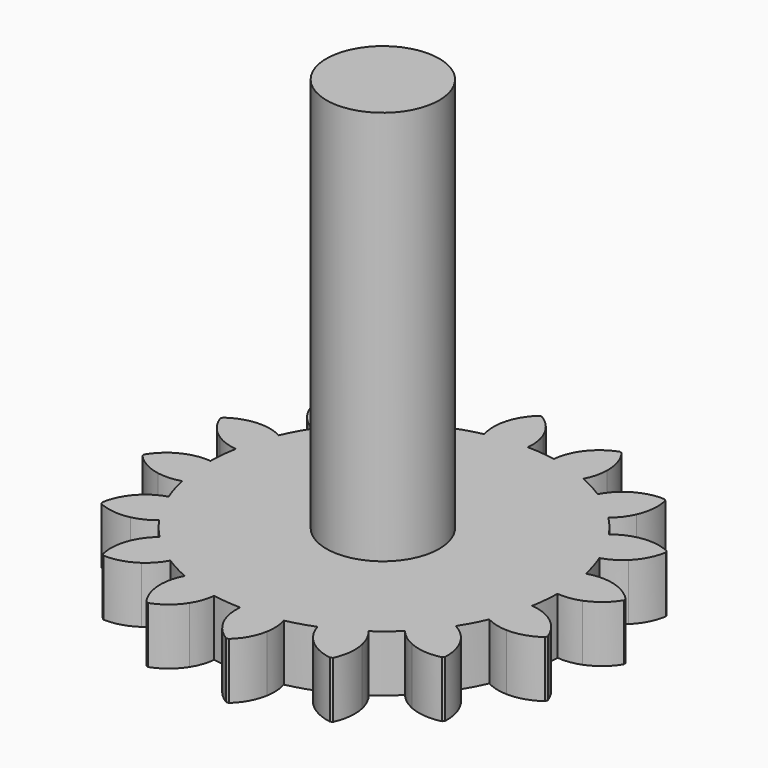
from build123d import *

# Parameters (mm, degrees)
F1_DEPTH = 1.5875
F2_COUNT = 16
F0_R     = 1.5875
F3_DEPTH = 1.5875
F4_DEPTH = 12.7


# Not quite as in the source:
# - a length typed as a fraction of an inch, garbled in the dataset ("3 / 203.2 mm" for 3/8 in), is restored


with BuildPart() as f1:
    # F0 (on Top) → F1 (new body)
    with BuildSketch(Plane.XY):
        with BuildLine():
            ThreePointArc((-1.051103421, 4.8804715195), (-0.4854789746, 4.9694364781), (0.0866333591, 4.9925288117))
            ThreePointArc((0.0866333591, 4.9925288117), (0.0808731678, 5.3155254225), (-7.85e-08, 5.6282865269))
            ThreePointArc((-7.85e-08, 5.6282865269), (-0.2339701384, 6.0238183846), (-0.5826076907, 6.3232166086))
            ThreePointArc((-0.5826076907, 6.3232166086), (-0.6185779348, 6.3208129001), (-0.6543259611, 6.3161529755))
            ThreePointArc((-0.6543259611, 6.3161529755), (-0.9378548446, 5.954491792), (-1.0901647979, 5.5209146738))
            ThreePointArc((-1.0901647979, 5.5209146738), (-1.108467423, 5.1983855986), (-1.051103421, 4.8804715195))
        make_face()
    extrude(amount=F1_DEPTH)


with BuildPart() as f2_1:
    # F2: instance of F1
    add(f1.part.rotate(Axis((-7.85e-08, 0.0402865269, 0), (0, 0, 1)), 1 * 360 / F2_COUNT))


with BuildPart() as f2_2:
    # F2: instance of F1
    add(f1.part.rotate(Axis((-7.85e-08, 0.0402865269, 0), (0, 0, 1)), 2 * 360 / F2_COUNT))


with BuildPart() as f2_3:
    # F2: instance of F1
    add(f1.part.rotate(Axis((-7.85e-08, 0.0402865269, 0), (0, 0, 1)), 3 * 360 / F2_COUNT))


with BuildPart() as f2_4:
    # F2: instance of F1
    add(f1.part.rotate(Axis((-7.85e-08, 0.0402865269, 0), (0, 0, 1)), 4 * 360 / F2_COUNT))


with BuildPart() as f2_5:
    # F2: instance of F1
    add(f1.part.rotate(Axis((-7.85e-08, 0.0402865269, 0), (0, 0, 1)), 5 * 360 / F2_COUNT))


with BuildPart() as f2_6:
    # F2: instance of F1
    add(f1.part.rotate(Axis((-7.85e-08, 0.0402865269, 0), (0, 0, 1)), 6 * 360 / F2_COUNT))


with BuildPart() as f2_7:
    # F2: instance of F1
    add(f1.part.rotate(Axis((-7.85e-08, 0.0402865269, 0), (0, 0, 1)), 7 * 360 / F2_COUNT))


with BuildPart() as f2_8:
    # F2: instance of F1
    add(f1.part.rotate(Axis((-7.85e-08, 0.0402865269, 0), (0, 0, 1)), 8 * 360 / F2_COUNT))


with BuildPart() as f2_9:
    # F2: instance of F1
    add(f1.part.rotate(Axis((-7.85e-08, 0.0402865269, 0), (0, 0, 1)), 9 * 360 / F2_COUNT))


with BuildPart() as f2_10:
    # F2: instance of F1
    add(f1.part.rotate(Axis((-7.85e-08, 0.0402865269, 0), (0, 0, 1)), 10 * 360 / F2_COUNT))


with BuildPart() as f2_11:
    # F2: instance of F1
    add(f1.part.rotate(Axis((-7.85e-08, 0.0402865269, 0), (0, 0, 1)), 11 * 360 / F2_COUNT))


with BuildPart() as f2_12:
    # F2: instance of F1
    add(f1.part.rotate(Axis((-7.85e-08, 0.0402865269, 0), (0, 0, 1)), 12 * 360 / F2_COUNT))


with BuildPart() as f2_13:
    # F2: instance of F1
    add(f1.part.rotate(Axis((-7.85e-08, 0.0402865269, 0), (0, 0, 1)), 13 * 360 / F2_COUNT))


with BuildPart() as f2_14:
    # F2: instance of F1
    add(f1.part.rotate(Axis((-7.85e-08, 0.0402865269, 0), (0, 0, 1)), 14 * 360 / F2_COUNT))


with BuildPart() as f2_15:
    # F2: instance of F1
    add(f1.part.rotate(Axis((-7.85e-08, 0.0402865269, 0), (0, 0, 1)), 15 * 360 / F2_COUNT))


with BuildPart() as f1_1:
    add(f1.part)

    add(f2_1.part)  # F3 merges F2_1

    add(f2_2.part)  # F3 merges F2_2

    add(f2_3.part)  # F3 merges F2_3

    add(f2_4.part)  # F3 merges F2_4

    add(f2_5.part)  # F3 merges F2_5

    add(f2_6.part)  # F3 merges F2_6

    add(f2_7.part)  # F3 merges F2_7

    add(f2_8.part)  # F3 merges F2_8

    add(f2_9.part)  # F3 merges F2_9

    add(f2_10.part)  # F3 merges F2_10

    add(f2_11.part)  # F3 merges F2_11

    add(f2_12.part)  # F3 merges F2_12

    add(f2_13.part)  # F3 merges F2_13

    add(f2_14.part)  # F3 merges F2_14

    add(f2_15.part)  # F3 merges F2_15
    # F0 (on Top) → F3 (join)
    with BuildSketch(Plane.XY):
        with BuildLine():
            ThreePointArc((-1.051103421, 4.8804715195), (-3.1085442832, -3.815768702), (4.9529999215, 0.0402865269))
            ThreePointArc((4.9529999215, 0.0402865269), (3.5327965769, 3.511821748), (0.0866333591, 4.9925288117))
            ThreePointArc((0.0866333591, 4.9925288117), (-0.4854789746, 4.9694364781), (-1.051103421, 4.8804715195))
        make_face()
        Circle(F0_R, mode=Mode.SUBTRACT)
    extrude(amount=F3_DEPTH)

    # F0 (on Top) → F4 (join)
    with BuildSketch(Plane.XY):
        Circle(F0_R)
    extrude(amount=F4_DEPTH)


solid = f1_1.part
